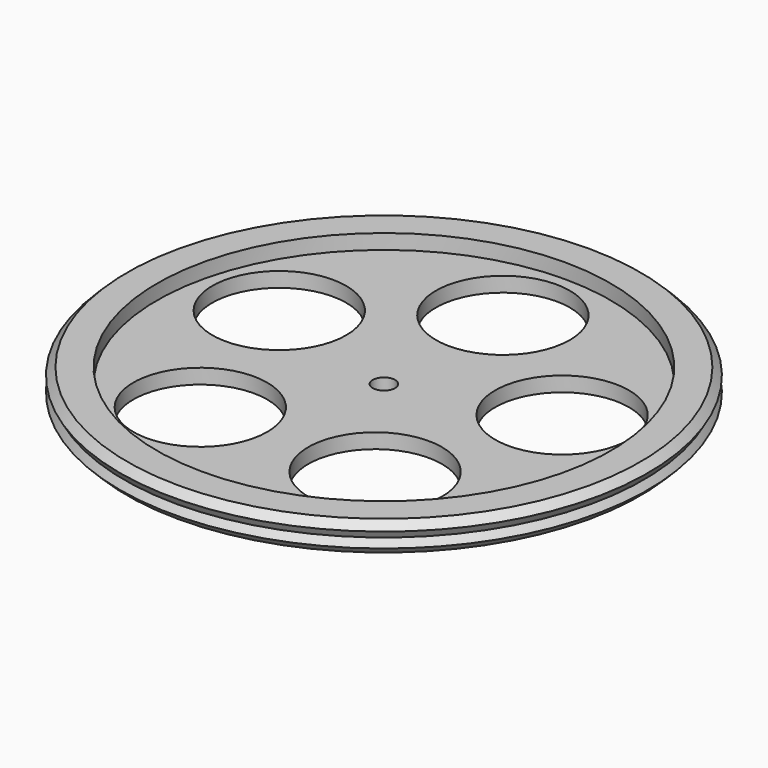
from build123d import *

# Parameters (mm, degrees)
F0_R     = 9
F0_R_2   = 1.5
F3_DEPTH = 25
F4_SIZE  = 0.99999


# Not quite as in the source:
# - a fillet or chamfer is up to 0.001 mm smaller than in the source, because OpenCascade refuses the exact size


with BuildPart() as f2:
    # F1 (on Right) → F2 (revolve)
    with BuildSketch(Plane.YZ):
        Polygon((0, 2), (0, 0), (35.5, 0), (35.5, 1), (34.9226497308, 2), (35.5, 3), (35.5, 4), (30.5, 4), (30.5, 2), align=None)
    revolve(axis=Axis((0, 0, 11.7082232609), (0, 0, 1)))

    # F0 (on Top) → F3 (cut)
    with BuildSketch(Plane.XY):
        with Locations((11.7557050458, -16.1803398875)):
            Circle(F0_R)
        with Locations((-11.7557050458, -16.1803398875)):
            Circle(F0_R)
        with Locations((-19.0211303259, 6.1803398875)):
            Circle(F0_R)
        with Locations((0, 20)):
            Circle(F0_R)
        with Locations((19.0211303259, 6.1803398875)):
            Circle(F0_R)
        Circle(F0_R_2)
    extrude(amount=F3_DEPTH, mode=Mode.SUBTRACT)

    # F4 (size 1 in the source; OpenCascade refuses exactly that, so slightly less here)
    f4_edges = [f2.edges().sort_by_distance(p)[0] for p in [
        (0, -35.5, 4),
        (0, -35.5, 0),
    ]]
    chamfer(f4_edges, length=F4_SIZE)


solid = f2.part
